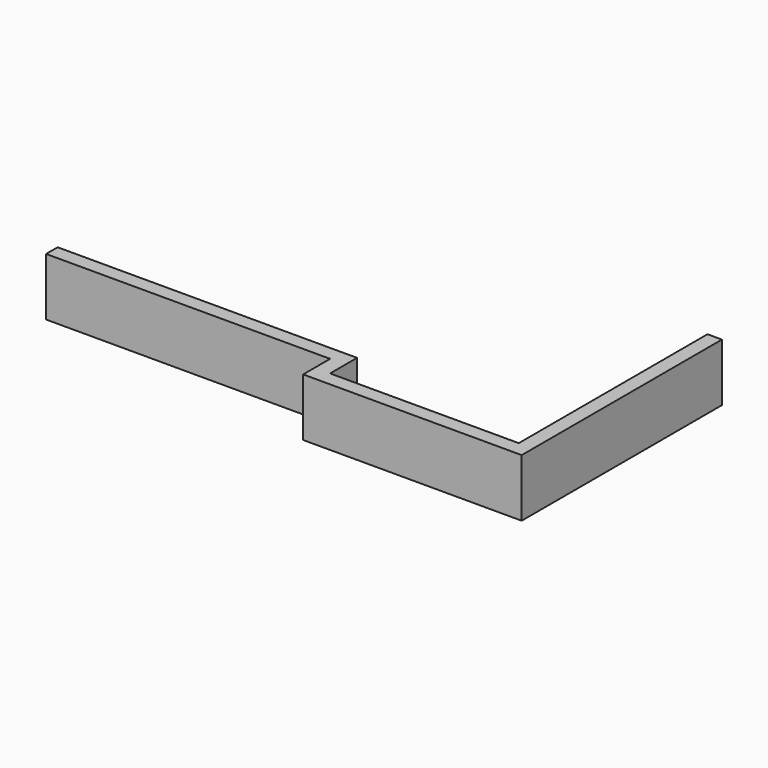
from build123d import *

# Parameters (mm, degrees)
F1_DEPTH = 76.2


# Not quite as in the source:
# - a feature names something its author has since deleted; it is built from what else it names


with BuildPart() as f1:
    # F0 (on Top) → F1 (new body)
    with BuildSketch(Plane.XY):
        Polygon((-190.23326214, -437.7922495125), (-190.23326214, -456.8422495125), (184.41673786, -456.8422495125), (184.41673786, -501.2922495125), (472.70673786, -501.2922495125), (472.70673786, -171.1285056541), (453.65673786, -171.1285056541), (453.65673786, -482.2785056541), (204.73673786, -482.2785056541), (204.73673786, -437.7559933709), (-172.45326214, -437.7559933709), align=None)
    extrude(amount=F1_DEPTH)


solid = f1.part
